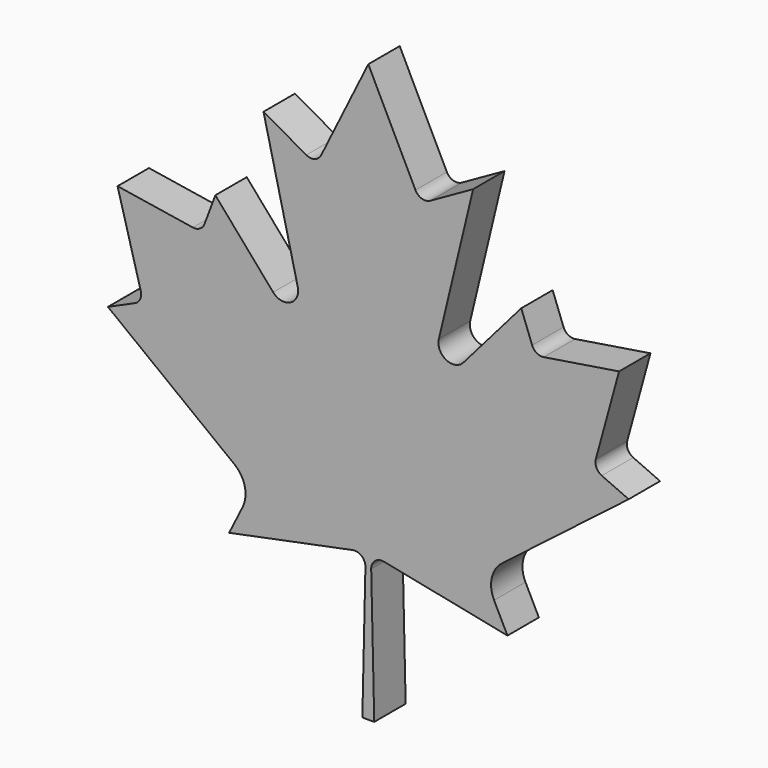
from build123d import *

# Parameters (mm, degrees)
F1_DEPTH = 1.4
F2_SCALE = 1.25


# Not quite as in the source:
# - ends of sketch curves that miss each other by under 0.0002 mm in the source are joined


with BuildPart() as f1:
    # F0 (on Front) → F1 (new body)
    with BuildSketch(Plane.XZ):
        with BuildLine():
            Line((2.0343041438, 15.7069808039), (0.3523669438, 19.1131970039))
            Line((0.3523669438, 19.1131970039), (0.3523669438, -1.4730457961))
            Line((0.3523669438, -1.4730457961), (0.5645331438, -1.4730457961))
            Line((0.5645331438, -1.4730457961), (0.4553893438, 3.2909274039))
            ThreePointArc((0.4553893438, 3.2909274039), (0.5916556183, 3.5917542423), (0.9117258932, 3.6731219434))
            Line((0.9117258932, 3.6731219434), (5.3169493438, 2.7830798039))
            Line((5.3169493438, 2.7830798039), (4.8399119438, 3.7367228039))
            ThreePointArc((4.8399119438, 3.7367228039), (4.7582554065, 4.4182578922), (5.1286096155, 4.9961801528))
            Line((5.1286096155, 4.9961801528), (9.6409691438, 8.4717908039))
            Line((9.6409691438, 8.4717908039), (8.6805951438, 8.9006952039))
            ThreePointArc((8.6805951438, 8.9006952039), (8.4915257857, 9.0857200238), (8.4685111742, 9.3492575516))
            Line((8.4685111742, 9.3492575516), (9.2975103438, 12.3747294039))
            Line((9.2975103438, 12.3747294039), (6.6119175438, 11.9498382039))
            ThreePointArc((6.6119175438, 11.9498382039), (6.3606002996, 11.996951044), (6.1956594084, 12.1923309026))
            Line((6.1956594084, 12.1923309026), (5.8086171438, 13.2239784039))
            Line((5.8086171438, 13.2239784039), (3.7461117438, 10.8478846039))
            ThreePointArc((3.7461117438, 10.8478846039), (3.1301426273, 10.7291430881), (2.8684469448, 11.2992470593))
            Line((2.8684469448, 11.2992470593), (4.0912977438, 16.4041346039))
            Line((4.0912977438, 16.4041346039), (2.5628527438, 15.5436588039))
            ThreePointArc((2.5628527438, 15.5436588039), (2.2634525656, 15.511644492), (2.0343041438, 15.7069808039))
        make_face()
        with BuildLine():
            Line((0.3523669438, -1.4730457961), (0.3523669438, 19.1131970039))
            Line((0.3523669438, 19.1131970039), (-1.3295956562, 15.7069808039))
            ThreePointArc((-1.3295956562, 15.7069808039), (-1.5587335044, 15.5116477594), (-1.858122509, 15.5436523149))
            Line((-1.858122509, 15.5436523149), (-3.3865892562, 16.4041346039))
            Line((-3.3865892562, 16.4041346039), (-2.1637316562, 11.2992426039))
            ThreePointArc((-2.1637316562, 11.2992426039), (-2.4254367706, 10.7291417351), (-3.0413892842, 10.8478967322))
            Line((-3.0413892842, 10.8478967322), (-5.1039086562, 13.2239784039))
            Line((-5.1039086562, 13.2239784039), (-5.4909284562, 12.1923320039))
            ThreePointArc((-5.4909284562, 12.1923320039), (-5.6558664119, 11.996951044), (-5.9071825723, 11.9498450545))
            Line((-5.9071825723, 11.9498450545), (-8.5927764562, 12.3747294039))
            Line((-8.5927764562, 12.3747294039), (-7.7637966562, 9.3492592039))
            ThreePointArc((-7.7637966562, 9.3492592039), (-7.786817298, 9.0857200238), (-7.9758860019, 8.9006937389))
            Line((-7.9758860019, 8.9006937389), (-8.9362606562, 8.4717908039))
            Line((-8.9362606562, 8.4717908039), (-4.4238744562, 4.9961818039))
            ThreePointArc((-4.4238744562, 4.9961818039), (-4.0535446709, 4.4182480852), (-4.1352063244, 3.7367242387))
            Line((-4.1352063244, 3.7367242387), (-4.6122408562, 2.7830798039))
            Line((-4.6122408562, 2.7830798039), (-0.2070172562, 3.6731212039))
            ThreePointArc((-0.2070172562, 3.6731212039), (0.1130528694, 3.5917542423), (0.2493205388, 3.2909273719))
            Line((0.2493205388, 3.2909273719), (0.1401753438, -1.4730457961))
            Line((0.1401753438, -1.4730457961), (0.3523669438, -1.4730457961))
        make_face()
    extrude(amount=F1_DEPTH)


with BuildPart() as f1_1:
    # F2: moved
    add(f1.part.scale(F2_SCALE).moved(Location((-0.088091736, 0.35, -4.778299251))))


solid = f1_1.part
